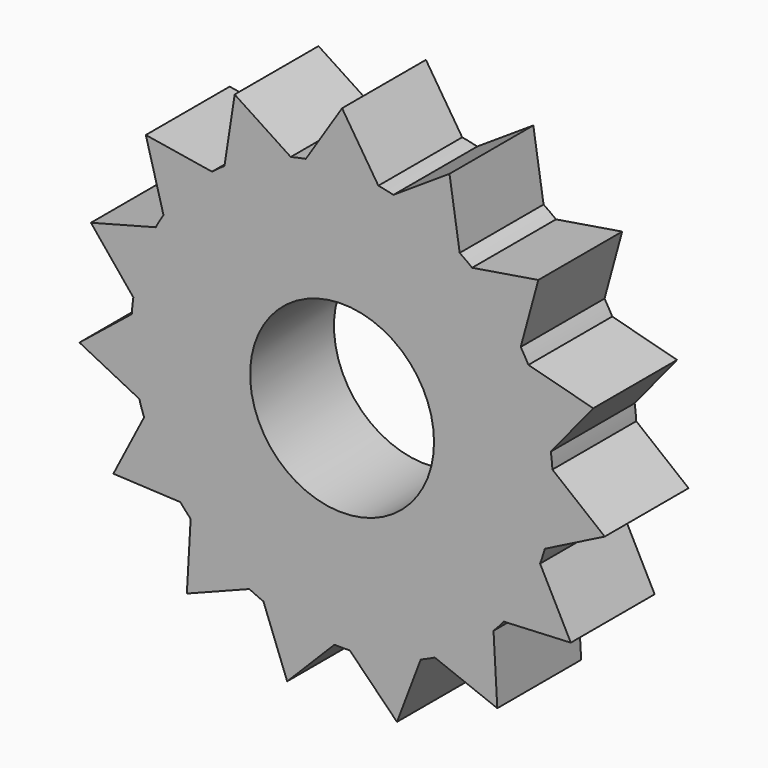
from build123d import *

# Parameters (mm, degrees)
F0_R            = 50.2948420816
F1_DEPTH        = 25
F2_R            = 21.9350719346
F3_DEPTH        = 25
F5_DEPTH        = 25
F5_COPIES_COUNT = 15


# Not quite as in the source:
# - a pattern or mirror of a feature is missing from the dataset's text; its kind, count and spacing are read off the source's solid


with BuildPart() as f1:
    # F0 (on Front) → F1 (new body)
    with BuildSketch(Plane.XZ):
        Circle(F0_R)
    extrude(amount=F1_DEPTH)

    # F2 (on face) → F3 (cut)
    with BuildSketch(Plane.XZ.offset(25)):
        Circle(F2_R)
    extrude(amount=-F3_DEPTH, mode=Mode.SUBTRACT)

    # F4 (on Front) → F5 (join)
    with BuildSketch(Plane.XZ):
        with BuildLine():
            Line((0, 63), (-8.656896714, 49.5442153969))
            ThreePointArc((-8.656896714, 49.5442153969), (0, 50.2948420816), (8.656896714, 49.5442153969))
            Line((8.656896714, 49.5442153969), (0, 63))
        make_face()
    f5 = extrude(amount=F5_DEPTH)

    # F5_copies: F5 ×15 about axis
    f5_copies_axis = Axis((0, 0, 0), (0, 1, 0))
    for i in range(1, F5_COPIES_COUNT):
        add(f5.rotate(f5_copies_axis, i * 360 / F5_COPIES_COUNT))


solid = f1.part
